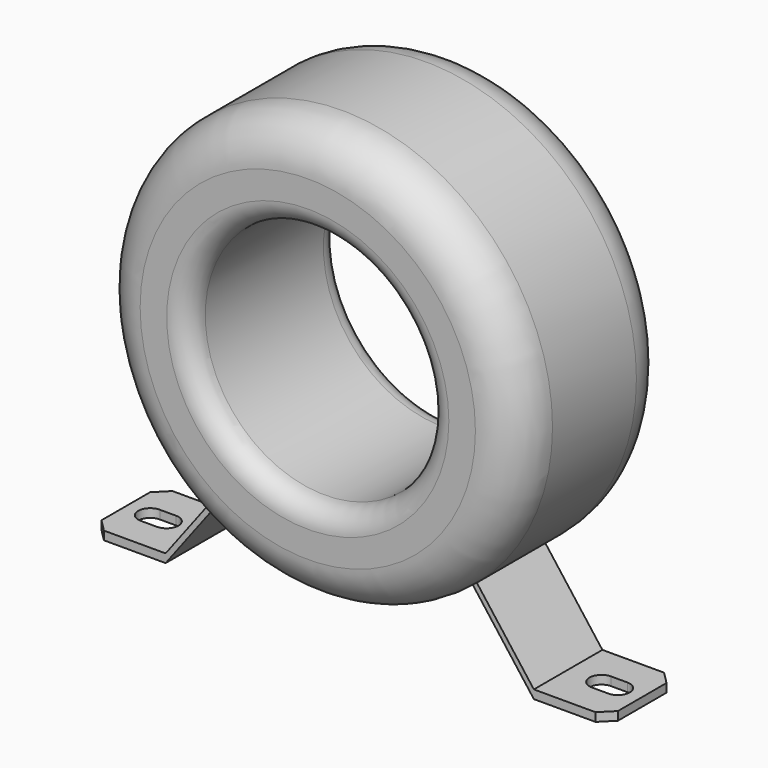
from build123d import *

# Parameters (mm, degrees)
F0_R     = 49.15
F0_R_2   = 27.95
F1_DEPTH = 22.25
F2_R     = 10
F3_R     = 5
F7_DEPTH = 2
F9_DEPTH = 20


with BuildPart() as f1:
    # F0 (on Front) → F1 (new body, symmetric)
    with BuildSketch(Plane.XZ):
        with Locations((0, 49.15)):
            Circle(F0_R)
        with Locations((0, 49.15)):
            Circle(F0_R_2, mode=Mode.SUBTRACT)
    extrude(amount=F1_DEPTH, both=True)

    # F2
    f2_edges = [f1.edges().sort_by_distance(p)[0] for p in [
        (-49.15, -22.25, 49.15),
        (-49.15, 22.25, 49.15),
    ]]
    fillet(f2_edges, radius=F2_R)

    # F3
    f3_edges = [f1.edges().sort_by_distance(p)[0] for p in [
        (-27.95, 22.25, 49.15),
        (-27.95, -22.25, 49.15),
    ]]
    fillet(f3_edges, radius=F3_R)



with BuildPart() as f7:
    # F5 (on face) → F7 (new body)
    with BuildSketch(Plane(origin=(0, 0, -9.7), x_dir=(1, 0, 0), z_dir=(0, 0, -1))):
        Polygon((43, 10), (43, -10), (57.4, -10), (60.3, -7.1), (60.3, 7.1), (57.4, 10), align=None)
        with BuildLine():
            ThreePointArc((54.6, 2.8), (56.5798989873, 1.9798989873), (57.4, 0))
            ThreePointArc((57.4, 0), (56.5798989873, -1.9798989873), (54.6, -2.8))
            Line((54.6, -2.8), (50.8, -2.8))
            ThreePointArc((50.8, -2.8), (48, 0), (50.8, 2.8))
            Line((50.8, 2.8), (54.6, 2.8))
        make_face(mode=Mode.SUBTRACT)
    extrude(amount=-F7_DEPTH)


with BuildPart() as f7b:
    # F5 (on face) → F7, piece 2 (new body)
    with BuildSketch(Plane(origin=(0, 0, -9.7), x_dir=(1, 0, 0), z_dir=(0, 0, -1))):
        Polygon((-57.4, -10), (-43, -10), (-43, 10), (-57.4, 10), (-60.3, 7.1), (-60.3, -7.1), align=None)
        with BuildLine():
            ThreePointArc((-54.6, -2.8), (-57.4, 0), (-54.6, 2.8))
            Line((-54.6, 2.8), (-50.8, 2.8))
            ThreePointArc((-50.8, 2.8), (-48.8201010127, 1.9798989873), (-48, 0))
            ThreePointArc((-48, 0), (-48.8201010127, -1.9798989873), (-50.8, -2.8))
            Line((-50.8, -2.8), (-54.6, -2.8))
        make_face(mode=Mode.SUBTRACT)
    extrude(amount=-F7_DEPTH)


with BuildPart() as f1_1:
    add(f1.part)

    add(f7.part)  # F9 merges F7

    add(f7b.part)  # F9 merges F7b
    # F8 (on face) → F9 (join, through all)
    with BuildSketch(Plane(origin=(0, 10, 0), x_dir=(-1, 0, 0), z_dir=(0, 1, 0))):
        with BuildLine():
            Line((43, -7.7), (29.6497265558, 9.9503033791))
            ThreePointArc((29.6497265558, 9.9503033791), (29.1663333729, 9.5893187927), (28.6785456751, 9.2342948458))
            Line((28.6785456751, 9.2342948458), (43, -9.7))
            Line((43, -9.7), (43, -7.7))
        make_face()
        with BuildLine():
            ThreePointArc((-28.6785456751, 9.2342948458), (-29.1663333729, 9.5893187927), (-29.6497265558, 9.9503033791))
            Line((-29.6497265558, 9.9503033791), (-43, -7.7))
            Line((-43, -7.7), (-43, -9.7))
            Line((-43, -9.7), (-28.6785456751, 9.2342948458))
        make_face()
    extrude(amount=-F9_DEPTH)


solid = f1_1.part
